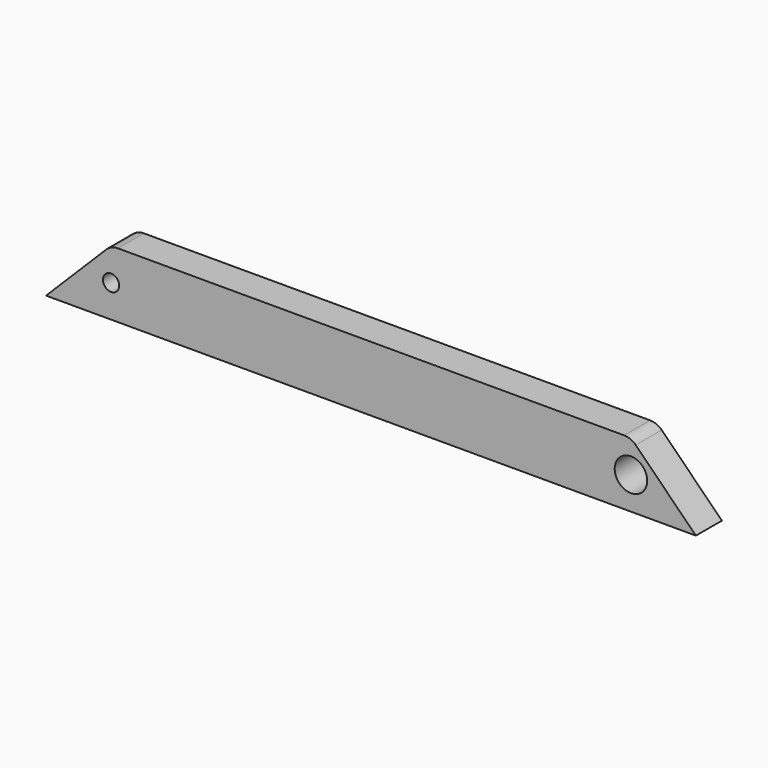
from build123d import *

# Parameters (mm, degrees)
F0_W     = 200
F0_H     = 20
F0_R     = 2.5
F0_R_2   = 5
F1_DEPTH = 5
F2_SIZE  = 19.99999
F3_R     = 5


# Not quite as in the source:
# - a fillet or chamfer is up to 0.001 mm smaller than in the source, because OpenCascade refuses the exact size


with BuildPart() as f1:
    # F0 (on Front) → F1 (new body, symmetric)
    with BuildSketch(Plane.XZ):
        with Locations((25, -13.3771840364)):
            Rectangle(F0_W, F0_H)
        with Locations((-55, -13.3771840364)):
            Circle(F0_R, mode=Mode.SUBTRACT)
        with Locations((105, -13.3771840364)):
            Circle(F0_R_2, mode=Mode.SUBTRACT)
    extrude(amount=F1_DEPTH, both=True)

    # F2 (size 20 in the source; OpenCascade refuses exactly that, so slightly less here)
    f2_edges = [f1.edges().sort_by_distance(p)[0] for p in [
        (-75, 0, -3.377184),
        (125, 0, -3.377184),
    ]]
    chamfer(f2_edges, length=F2_SIZE)

    # F3
    f3_edges = [f1.edges().sort_by_distance(p)[0] for p in [
        (-55.00001, 0, -3.377184),
        (105.00001, 0, -3.377184),
    ]]
    fillet(f3_edges, radius=F3_R)


solid = f1.part
